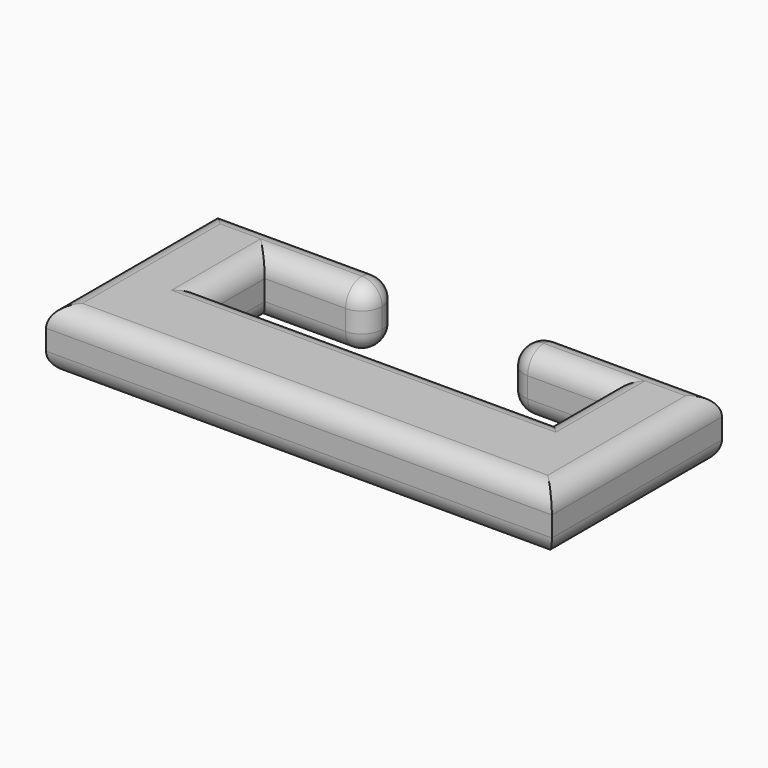
from build123d import *

# Parameters (mm, degrees)
F0_W     = 12.7
F0_H     = 5.08
F1_DEPTH = 7.62
F2_R     = 2.53999


# Not quite as in the source:
# - a fillet or chamfer is up to 0.001 mm smaller than in the source, because OpenCascade refuses the exact size


with BuildPart() as f1:
    # F0 (on Top) → F1 (new body)
    with BuildSketch(Plane.XY):
        Polygon((-30.1547096223, 19.9307221919), (-30.1547096223, 5.9384261601), (-19.9947096223, 5.9384261601), (-19.9947096223, 14.8507221919), (-19.9947096223, 19.9307221919), align=None)
        Polygon((-19.9947096223, 5.9384261601), (-30.1547096223, 5.9384261601), (-30.1547096223, -6.7615738399), (33.3452903777, -6.7615738399), (33.3452903777, 5.9384261601), (23.1852903777, 5.9384261601), align=None)
        Polygon((23.1852903777, 14.8507221919), (23.1852903777, 5.9384261601), (33.3452903777, 5.9384261601), (33.3452903777, 19.9307221919), (23.1852903777, 19.9307221919), align=None)
        with Locations((-13.6447096223, 17.3907221919)):
            Rectangle(F0_W, F0_H)
        with Locations((16.8352903777, 17.3907221919)):
            Rectangle(F0_W, F0_H)
    extrude(amount=F1_DEPTH)

    # F2 (radius 2.54 in the source; OpenCascade refuses exactly that, so slightly less here)
    f2_edges = [f1.edges().sort_by_distance(p)[0] for p in [
        (1.59529, -6.761574, 7.62),
        (1.59529, 5.938426, 7.62),
        (-30.15471, 6.584574, 7.62),
        (33.34529, 6.584574, 7.62),
        (21.91529, 19.930722, 7.62),
        (-18.72471, 19.930722, 7.62),
        (21.91529, 19.930722, 0),
        (23.18529, 10.394574, 7.62),
        (16.83529, 14.850722, 7.62),
        (-13.64471, 14.850722, 7.62),
        (1.59529, -6.761574, 0),
        (-30.15471, 6.584574, 0),
        (33.34529, 6.584574, 0),
        (10.48529, 14.850722, 3.81),
        (10.48529, 19.930722, 3.81),
        (-7.29471, 14.850722, 3.81),
        (-7.29471, 19.930722, 3.81),
        (-19.99471, 10.394574, 7.62),
        (1.59529, 5.938426, 0),
        (-19.99471, 10.394574, 0),
        (16.83529, 14.850722, 0),
        (23.18529, 10.394574, 0),
        (-13.64471, 14.850722, 0),
        (10.48529, 17.390722, 0),
        (-7.29471, 17.390722, 0),
        (-18.72471, 19.930722, 0),
        (10.48529, 17.390722, 7.62),
        (-7.29471, 17.390722, 7.62),
    ]]
    fillet(f2_edges, radius=F2_R)


solid = f1.part
